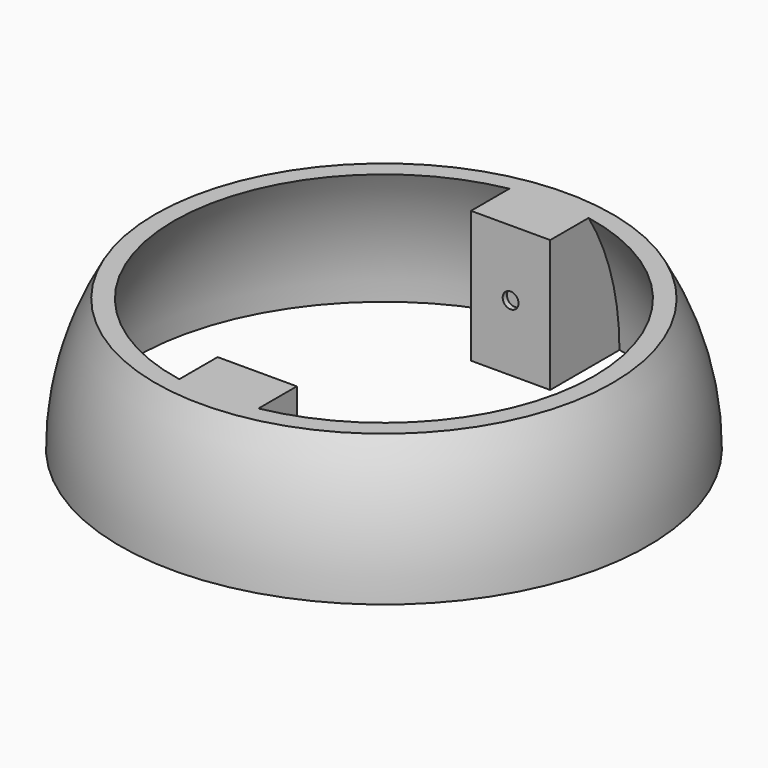
from build123d import *

# Parameters (mm, degrees)
F2_T     = -6
F4_W     = 30
F4_H     = 50
F6_R     = 3
F7_DEPTH = 2


# Not quite as in the source:
# - a pattern or mirror of a feature is missing from the dataset's text; its kind, count and spacing are read off the source's solid


with BuildPart() as f1:
    # F0 (on Front) → F1 (revolve)
    with BuildSketch(Plane.XZ):
        with BuildLine():
            Line((0, 50), (-86.6025403784, 50))
            ThreePointArc((-86.6025403784, 50), (-96.5925826289, 25.8819045103), (-100, 0))
            Line((-100, 0), (0, 0))
            Line((0, 0), (0, 50))
        make_face()
    revolve(axis=Axis((0, 0, 25), (0, 0, -1)))

    # F2
    f2_openings = [f1.faces().sort_by_distance(p)[0] for p in [
        (0, 0, 50),
        (0, 0, 0),
    ]]
    offset(amount=F2_T, openings=f2_openings)

    # F4 (on offset) → F5 (join, up to the next surface of F1)
    with BuildSketch(Plane.XZ.offset(-60)):
        with Locations((0, 25)):
            Rectangle(F4_W, F4_H)
    f5 = extrude(until=Until.NEXT, dir=(0, 1, 0))

    # F5_copies: F5 across plane
    add(f5.mirror(Plane(origin=(0, 0, 0), x_dir=(0, 0, -1), z_dir=(0, -1, 0))))

    # F6 (on face) → F7 (cut)
    with BuildSketch(Plane.XZ.offset(-60)):
        with Locations((0, 25)):
            Circle(F6_R)
    f7 = extrude(amount=-F7_DEPTH, mode=Mode.SUBTRACT)

    # F7_copies: F7 across plane
    add(f7.mirror(Plane(origin=(0, 0, 0), x_dir=(0, 0, -1), z_dir=(0, -1, 0))), mode=Mode.SUBTRACT)


solid = f1.part
